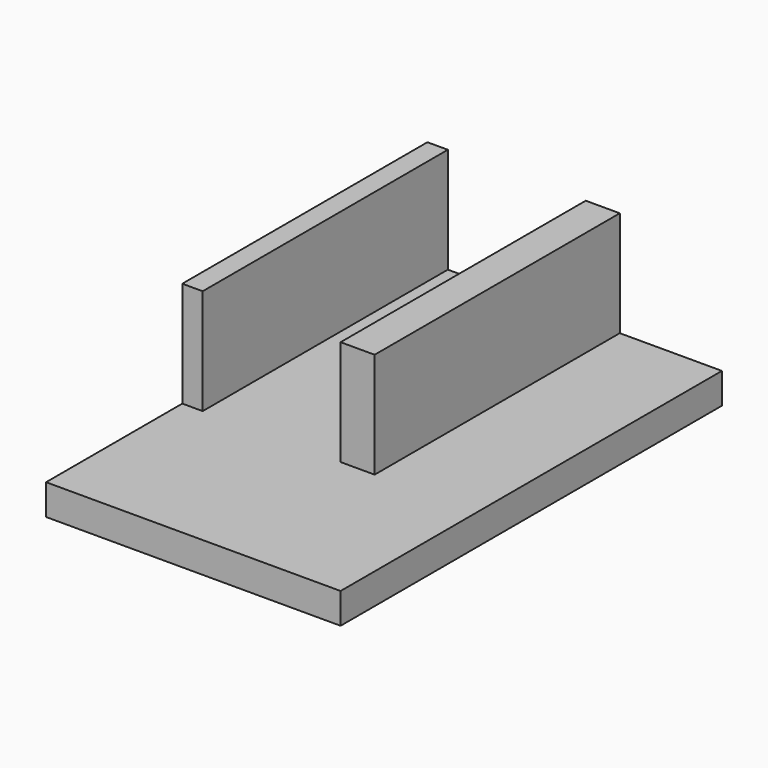
from build123d import *

# Parameters (mm, degrees)
F0_W     = 8.1
F0_H     = 18
F1_DEPTH = 1.8
F0_W_2   = 1.2
F0_W_3   = 2
F2_DEPTH = 8


# Not quite as in the source:
# - a feature names something its author has since deleted; it is built from what else it names


with BuildPart() as f1:
    # F0 (on Top) → F1 (new body)
    with BuildSketch(Plane.XY):
        Polygon((6.05, -9), (4.05, -9), (-4.05, -9), (-5.25, -9), (-5.25, -19), (6.05, -19), align=None)
        Rectangle(F0_W, F0_H)
        Polygon((6.05, 9), (6.05, -9), (6.05, -19), (12.05, -19), (12.05, 9), align=None)
    extrude(amount=F1_DEPTH)

    # F0 (on Top) → F2 (join)
    with BuildSketch(Plane.XY):
        with Locations((-4.65, 0)):
            Rectangle(F0_W_2, F0_H)
        with Locations((5.05, 0)):
            Rectangle(F0_W_3, F0_H)
    extrude(amount=F2_DEPTH)


solid = f1.part
